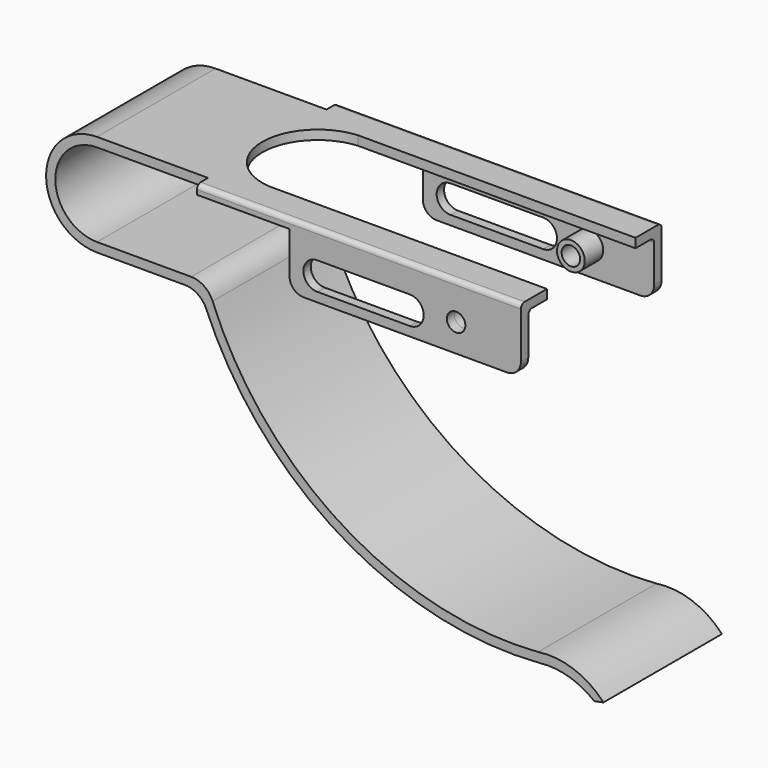
from build123d import *

# Parameters (mm, degrees)
F1_DEPTH  = 16
F3_W      = 70
F3_H      = 3
F4_DEPTH  = 2
F5_W      = 50
F5_H      = 14
F6_DEPTH  = 2
F7_R      = 1
F10_DEPTH = 2
F12_DEPTH = 38.001
F14_D     = 4
F15_R     = 3
F15_R_2   = 2
F16_DEPTH = 5
F17_R     = 3


# Not quite as in the source:
# - a pattern or mirror of a feature is missing from the dataset's text; its kind, count and spacing are read off the source's solid


with BuildPart() as f1:
    # F0 (on Front) → F1 (new body)
    with BuildSketch(Plane.XZ):
        with BuildLine():
            ThreePointArc((0, -9), (-9, 0), (0, 9))
            Line((0, 9), (94, 9))
            Line((94, 9), (94, 11))
            Line((94, 11), (0, 11))
            ThreePointArc((0, 11), (-11, 0), (0, -11))
            Line((0, -11), (19, -11))
            ThreePointArc((19, -11), (21.7681124643, -11.8361612201), (23.6103896104, -14.064978646))
            ThreePointArc((23.6103896104, -14.064978646), (52.4527960943, -47.6352500016), (95.4829432523, -57.9915990802))
            ThreePointArc((95.4829432523, -57.9915990802), (101.8289994783, -58.4789828394), (107.4829432523, -61.4018055084))
            Line((107.4829432523, -61.4018055084), (109.4421656321, -61))
            ThreePointArc((109.4421656321, -61), (102.9917579834, -56.7391896111), (95.2965735981, -56))
            ThreePointArc((95.2965735981, -56), (52.955209083, -45.5949761441), (24.9861322889, -12.1467114099))
            ThreePointArc((24.9861322889, -12.1467114099), (23.1470623984, -9.8607704249), (20.3422845953, -9))
            Line((20.3422845953, -9), (0, -9))
        make_face()
    extrude(amount=F1_DEPTH)

    # F3 (on face) → F4 (join)
    with BuildSketch(Plane.XY.offset(11)):
        with Locations((59, -17.5)):
            Rectangle(F3_W, F3_H)
    extrude(amount=-F4_DEPTH)

    # F5 (on face) → F6 (join)
    with BuildSketch(Plane.XZ.offset(19)):
        with Locations((69, 4)):
            Rectangle(F5_W, F5_H)
    extrude(amount=-F6_DEPTH)

    # F7
    f7_edges = [f1.edges().sort_by_distance(p)[0] for p in [
        (59, -19, 11),
        (69, -17, 9),
    ]]
    fillet(f7_edges, radius=F7_R)

    # F8: F1 across plane


with BuildPart() as f1_1:
    add(f1.part)
    add(f1.part.mirror(Plane.XZ))

    # F9 (on face) → F10 (cut)
    with BuildSketch(Plane.XY.offset(11)):
        with BuildLine():
            Line((94, 11.964731734), (34, 11.964731734))
            ThreePointArc((34, 11.964731734), (22.9193446211, 0), (34, -11.964731734))
            Line((34, -11.964731734), (94, -11.964731734))
            Line((94, -11.964731734), (94, 11.964731734))
        make_face()
    extrude(amount=-F10_DEPTH, mode=Mode.SUBTRACT)

    # F11 (on face) → F12 (cut, through all)
    with BuildSketch(Plane.XZ.offset(19)):
        with BuildLine():
            ThreePointArc((50, 5), (47, 2), (50, -1))
            Line((50, -1), (70, -1))
            ThreePointArc((70, -1), (73, 2), (70, 5))
            Line((70, 5), (50, 5))
        make_face()
    extrude(amount=-F12_DEPTH, mode=Mode.SUBTRACT)

    # F14 (through all)
    with Locations(Plane.XZ.offset(19)):
        with Locations((80, 3)):
            Hole(F14_D / 2)

    # F15 (on face) → F16 (join)
    with BuildSketch(Plane(origin=(0, -17, 0), x_dir=(-1, 0, 0), z_dir=(0, 1, 0))):
        with Locations((-80, 3)):
            Circle(F15_R)
        with Locations((-80, 3)):
            Circle(F15_R_2, mode=Mode.SUBTRACT)
    f16 = extrude(amount=F16_DEPTH)

    # F16_copies: F16 across plane
    add(f16.mirror(Plane.ZX))

    # F17
    f17_edges = [f1_1.edges().sort_by_distance(p)[0] for p in [
        (44, -18, -3),
        (94, 18, -3),
        (94, -18, -3),
        (44, 18, -3),
    ]]
    fillet(f17_edges, radius=F17_R)


solid = f1_1.part
